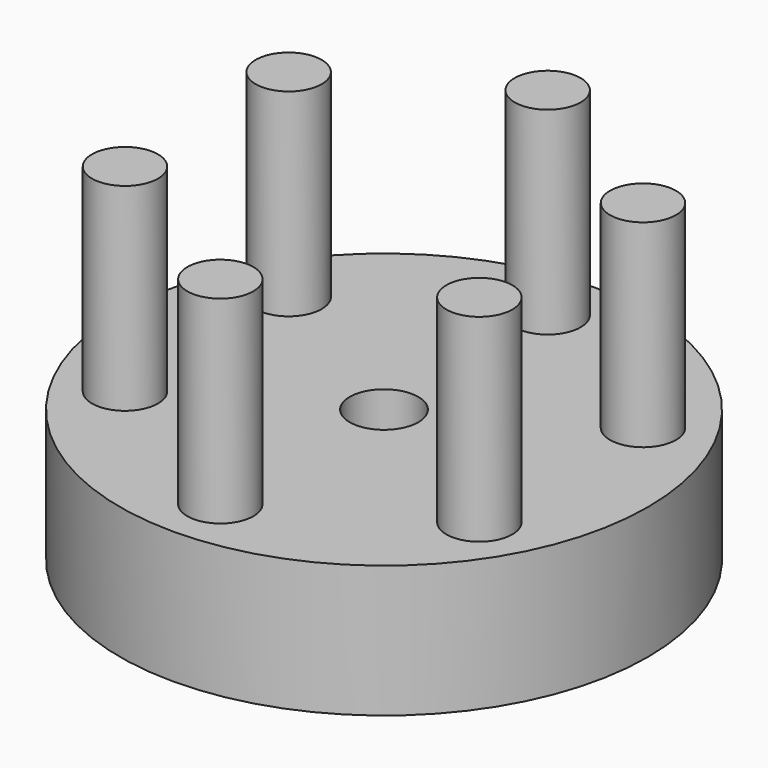
from build123d import *

# Parameters (mm, degrees)
F0_R     = 25.4
F1_DEPTH = 12.7
F2_R     = 3.302
F3_DEPTH = 12.7
F4_R     = 3.175
F5_DEPTH = 19.05


# Not quite as in the source:
# - a feature names something its author has since deleted; it is built from what else it names


with BuildPart() as f1:
    # F0 (on Top) → F1 (new body)
    with BuildSketch(Plane.XY):
        Circle(F0_R)
    extrude(amount=F1_DEPTH)

    # F2 (on face) → F3 (cut)
    with BuildSketch(Plane(origin=(0, 0, 0), x_dir=(1, 0, 0), z_dir=(0, 0, -1))):
        Circle(F2_R)
    extrude(amount=-F3_DEPTH, mode=Mode.SUBTRACT)

    # F4 (on face) → F5 (join)
    with BuildSketch(Plane.XY.offset(12.7)):
        with Locations((0, 19.685)):
            Circle(F4_R)
        with Locations((-17.0477100735, 9.8425)):
            Circle(F4_R)
        with Locations((-17.0477100735, -9.8425)):
            Circle(F4_R)
        with Locations((0, -19.685)):
            Circle(F4_R)
        with Locations((17.0477100735, -9.8425)):
            Circle(F4_R)
        with Locations((17.0477100735, 9.8425)):
            Circle(F4_R)
    extrude(amount=F5_DEPTH)


solid = f1.part
